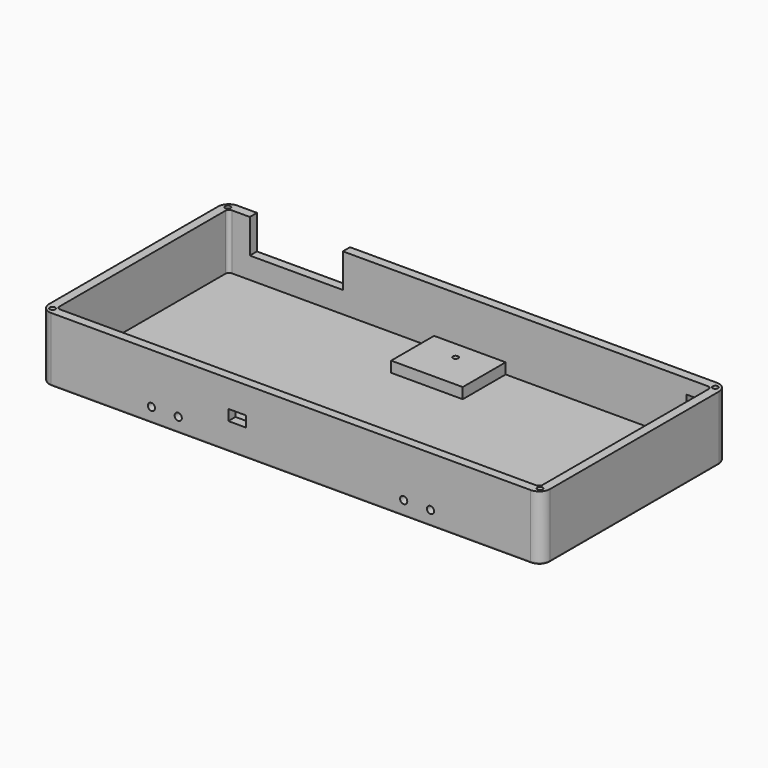
from build123d import *

# Parameters (mm, degrees)
F0_W      = 280
F0_H      = 130
F1_DEPTH  = 36
F2_W      = 270
F2_H      = 120
F3_DEPTH  = 31
F4_R      = 2
F4_W      = 10
F4_H      = 6
F6_DEPTH  = 25
F5_W      = 52
F5_H      = 19
F5_W_2    = 9
F5_H_2    = 11
F7_DEPTH  = 25
F8_W      = 40
F8_H      = 30
F9_DEPTH  = 11
F10_R     = 1.5
F11_DEPTH = 12
F12_R     = 1.5
F13_DEPTH = 12
F14_R     = 6
F15_R     = 2
F16_R     = 1


# Not quite as in the source:
# - a feature names something its author has since deleted; it is built from what else it names


with BuildPart() as f1:
    # F0 (on Top) → F1 (new body)
    with BuildSketch(Plane.XY):
        with Locations((-12.5971958935, -11.2710741152)):
            Rectangle(F0_W, F0_H)
    extrude(amount=F1_DEPTH)

    # F2 (on face) → F3 (cut)
    with BuildSketch(Plane.XY.offset(36)):
        with Locations((-12.5971958935, -11.2710741152)):
            Rectangle(F2_W, F2_H)
    extrude(amount=-F3_DEPTH, mode=Mode.SUBTRACT)

    # F4 (on face) → F6 (cut)
    with BuildSketch(Plane.XZ.offset(76.2710741152)):
        with Locations((-90.5971958935, 8)):
            Circle(F4_R)
        with Locations((-75.5971958935, 8)):
            Circle(F4_R)
        with Locations((50.4028041065, 8)):
            Circle(F4_R)
        with Locations((65.4028041065, 8)):
            Circle(F4_R)
        with Locations((-42.5971958935, 18)):
            Rectangle(F4_W, F4_H)
    extrude(amount=-F6_DEPTH, mode=Mode.SUBTRACT)

    # F5 (on face) → F7 (cut)
    with BuildSketch(Plane(origin=(0, 53.7289258848, 0), x_dir=(-1, 0, 0), z_dir=(0, 1, 0))):
        with Locations((109.5971958935, 26.5)):
            Rectangle(F5_W, F5_H)
        with Locations((-112.9028041065, 22.5)):
            Rectangle(F5_W_2, F5_H_2)
    extrude(amount=-F7_DEPTH, mode=Mode.SUBTRACT)

    # F8 (on face) → F9 (join)
    with BuildSketch(Plane(origin=(0, 0, 0), x_dir=(1, 0, 0), z_dir=(0, 0, -1))):
        with Locations((-12.5971958935, -33.7289258848)):
            Rectangle(F8_W, F8_H)
        with Locations((-12.5971958935, 56.2710741152)):
            Rectangle(F8_W, F8_H)
    extrude(amount=-F9_DEPTH)

    # F10 (on face) → F11 (cut)
    with BuildSketch(Plane.XY.offset(11)):
        with Locations((-12.5971958935, 38.7289258848)):
            Circle(F10_R)
        with Locations((-12.5971958935, -61.2710741152)):
            Circle(F10_R)
    extrude(amount=-F11_DEPTH, mode=Mode.SUBTRACT)

    # F12 (on face) → F13 (cut)
    with BuildSketch(Plane.XY.offset(36)):
        with Locations((-148.8471958935, 49.9789258848)):
            Circle(F12_R)
        with Locations((-148.8471958935, -72.5210741152)):
            Circle(F12_R)
        with Locations((123.6528041065, -72.5210741152)):
            Circle(F12_R)
        with Locations((123.6528041065, 49.9789258848)):
            Circle(F12_R)
    extrude(amount=-F13_DEPTH, mode=Mode.SUBTRACT)

    # F14
    f14_edges = [f1.edges().sort_by_distance(p)[0] for p in [
        (-152.597196, -76.271074, 18),
        (-152.597196, 53.728926, 18),
        (127.402804, -76.271074, 18),
        (127.402804, 53.728926, 18),
    ]]
    fillet(f14_edges, radius=F14_R)

    # F15
    f15_edges = [f1.edges().sort_by_distance(p)[0] for p in [
        (-147.597196, 48.728926, 20.5),
        (-147.597196, -71.271074, 20.5),
        (122.402804, 48.728926, 20.5),
        (122.402804, -71.271074, 20.5),
    ]]
    fillet(f15_edges, radius=F15_R)

    # F16
    f16_edges = [f1.edges().sort_by_distance(p)[0] for p in [
        (-152.597196, -11.271074, 0),
    ]]
    fillet(f16_edges, radius=F16_R)


solid = f1.part
